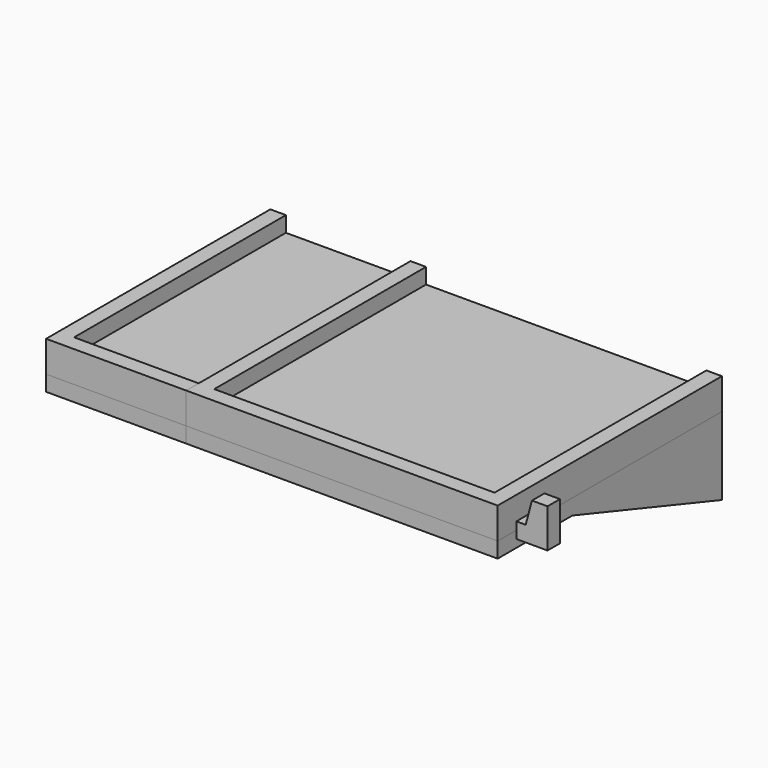
from build123d import *

# Parameters (mm, degrees)
F0_W      = 50.8
F0_H      = 101.6
F0_H_2    = 6.35
F1_DEPTH  = 6.35
F0_W_2    = 114.3
F0_W_3    = 6.35
F2_DEPTH  = 12.7
F3_DEPTH  = 12.7
F4_DEPTH  = 6.35
F5_DEPTH  = 6.35
F7_DEPTH  = 6.35
F9_DEPTH  = 6.35
F11_DEPTH = 12.7
F12_W     = 6.35
F12_H     = 6.35
F13_DEPTH = 9.525
F15_DEPTH = 6.35


# Not quite as in the source:
# - a feature names something its author has since deleted; it is built from what else it names


with BuildPart() as f1:
    # F0 (on Top) → F1 (new body)
    with BuildSketch(Plane.XY):
        with Locations((-88.9, 0)):
            Rectangle(F0_W, F0_H)
        with Locations((-88.9, 53.975)):
            Rectangle(F0_W, F0_H_2)
    extrude(amount=F1_DEPTH)


with BuildPart() as f1b:
    # F0 (on Top) → F1, piece 2 (new body)
    with BuildSketch(Plane.XY):
        Rectangle(F0_W_2, F0_H)
        with Locations((0, 53.975)):
            Rectangle(F0_W_2, F0_H_2)
    extrude(amount=F1_DEPTH)


with BuildPart() as f2:
    # F0 (on Top) → F2 (new body)
    with BuildSketch(Plane.XY):
        with Locations((-60.325, 53.975)):
            Rectangle(F0_W_3, F0_H_2)
        with Locations((-60.325, 0)):
            Rectangle(F0_W_3, F0_H)
        with Locations((-60.325, -53.975)):
            Rectangle(F0_W_3, F0_H_2)
        with Locations((0, -53.975)):
            Rectangle(F0_W_2, F0_H_2)
        with Locations((60.325, 0)):
            Rectangle(F0_W_3, F0_H)
        with Locations((60.325, 53.975)):
            Rectangle(F0_W_3, F0_H_2)
        with Locations((60.325, -53.975)):
            Rectangle(F0_W_3, F0_H_2)
    extrude(amount=F2_DEPTH)


with BuildPart() as f3:
    # F0 (on Top) → F3 (new body)
    with BuildSketch(Plane.XY):
        Polygon((-114.3, 50.8), (-114.3, 57.15), (-120.65, 57.15), (-120.65, -57.15), (-114.3, -57.15), (-114.3, -50.8), align=None)
        with Locations((-88.9, -53.975)):
            Rectangle(F0_W, F0_H_2)
    extrude(amount=F3_DEPTH)


with BuildPart() as f4:
    # F0 (on Top) → F4 (new body)
    with BuildSketch(Plane.XY):
        with Locations((-60.325, -53.975)):
            Rectangle(F0_W_3, F0_H_2)
        with Locations((0, -53.975)):
            Rectangle(F0_W_2, F0_H_2)
        with Locations((60.325, -53.975)):
            Rectangle(F0_W_3, F0_H_2)
        with Locations((60.325, 0)):
            Rectangle(F0_W_3, F0_H)
        with Locations((60.325, 53.975)):
            Rectangle(F0_W_3, F0_H_2)
    extrude(amount=-F4_DEPTH)

    # F6 (on face) → F7 (join)
    with BuildSketch(Plane.YZ.offset(63.5)):
        Polygon((57.15, -31.75), (57.15, -6.35), (-19.05, -6.35), align=None)
    extrude(amount=-F7_DEPTH)


with BuildPart() as f5:
    # F0 (on Top) → F5 (new body)
    with BuildSketch(Plane.XY):
        with Locations((-88.9, -53.975)):
            Rectangle(F0_W, F0_H_2)
        Polygon((-114.3, 50.8), (-114.3, 57.15), (-120.65, 57.15), (-120.65, -57.15), (-114.3, -57.15), (-114.3, -50.8), align=None)
    extrude(amount=-F5_DEPTH)


with BuildPart() as f9:
    # F8 (on face) → F9 (new body)
    with BuildSketch(Plane(origin=(-120.65, 0, 0), x_dir=(0, -1, 0), z_dir=(-1, 0, 0))):
        Polygon((19.05, -6.35), (-57.15, -6.35), (-57.15, -31.75), align=None)
    extrude(amount=-F9_DEPTH)


with BuildPart() as f11:
    # F10 (on face) → F11 (new body)
    with BuildSketch(Plane.YZ.offset(63.5)):
        Polygon((-47.625, 3.175), (-47.625, 0), (-44.45, 0), (-41.275, 0), (-41.275, 3.175), align=None)
        Polygon((-44.45, 0), (-47.625, 0), (-47.625, -3.175), (-41.275, -3.175), (-41.275, 0), align=None)
    extrude(amount=F11_DEPTH)

    # F12 (on face) → F13 (join)
    with BuildSketch(Plane.XY.offset(3.175)):
        with Locations((73.025, -44.45)):
            Rectangle(F12_W, F12_H)
    extrude(amount=F13_DEPTH)

    # F14 (on face) → F15 (join)
    with BuildSketch(Plane.XZ.offset(47.625)):
        Polygon((67.31, 3.175), (69.85, 3.175), (69.85, 12.7), align=None)
    extrude(amount=-F15_DEPTH)


solid = Compound([f1.part, f1b.part, f2.part, f3.part, f4.part, f5.part, f9.part, f11.part])
